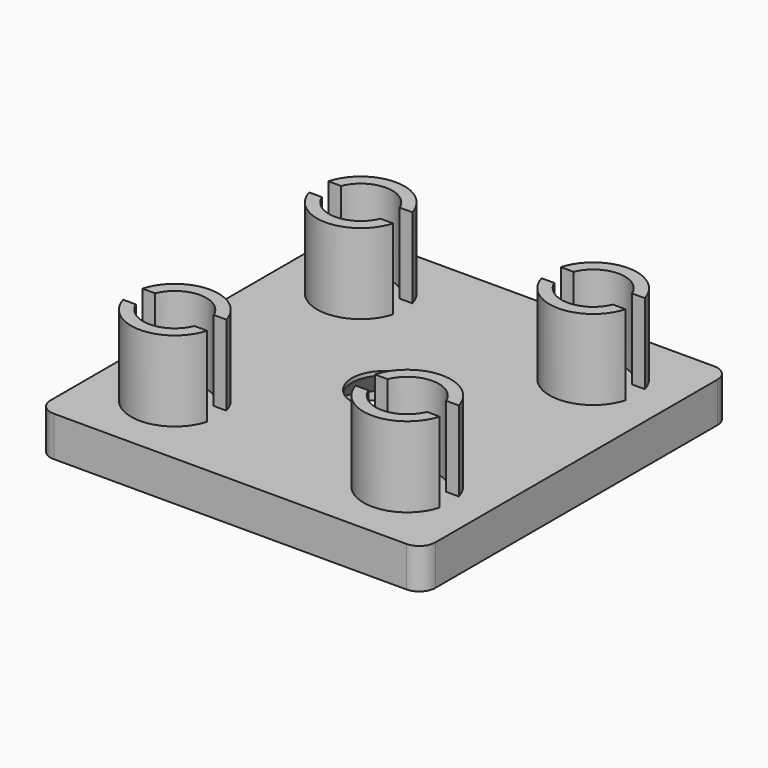
from build123d import *

# Parameters (mm, degrees)
F0_W           = 36
F0_H           = 36
F1_DEPTH       = 4
F3_DEPTH       = 10
F5_D           = 8
F5_CSINK_D     = 15
F5_CSINK_ANGLE = 90
F6_DEPTH       = 1


with BuildPart() as f1:
    # F0 (on Top) → F1 (new body)
    with BuildSketch(Plane.XY):
        with BuildLine():
            ThreePointArc((24, 22), (23.4142135624, 23.4142135624), (22, 24))
            Line((22, 24), (-22, 24))
            ThreePointArc((-22, 24), (-23.4142135624, 23.4142135624), (-24, 22))
            Line((-24, 22), (-24, -22))
            ThreePointArc((-24, -22), (-23.4142135624, -23.4142135624), (-22, -24))
            Line((-22, -24), (22, -24))
            ThreePointArc((22, -24), (23.4142135624, -23.4142135624), (24, -22))
            Line((24, -22), (24, 22))
        make_face()
        Rectangle(F0_W, F0_H, mode=Mode.SUBTRACT)
        Rectangle(F0_W, F0_H)
    extrude(amount=-F1_DEPTH)

    # F2 (on face) → F3 (join)
    with BuildSketch(Plane.XY):
        with BuildLine():
            Line((18.1541072781, 16), (19.7395133362, 16))
            ThreePointArc((19.7395133362, 16), (14.5, 19.95), (9.2604866638, 16))
            Line((9.2604866638, 16), (10.8458927219, 16))
            ThreePointArc((10.8458927219, 16), (14.5, 18.45), (18.1541072781, 16))
        make_face()
        with BuildLine():
            ThreePointArc((9.2604866638, 13), (14.5, 9.05), (19.7395133362, 13))
            Line((19.7395133362, 13), (18.1541072781, 13))
            ThreePointArc((18.1541072781, 13), (14.5, 10.55), (10.8458927219, 13))
            Line((10.8458927219, 13), (9.2604866638, 13))
        make_face()
        with BuildLine():
            Line((-10.8458927219, 16), (-9.2604866638, 16))
            ThreePointArc((-9.2604866638, 16), (-14.5, 19.95), (-19.7395133362, 16))
            Line((-19.7395133362, 16), (-18.1541072781, 16))
            ThreePointArc((-18.1541072781, 16), (-14.5, 18.45), (-10.8458927219, 16))
        make_face()
        with BuildLine():
            ThreePointArc((-19.7395133362, 13), (-14.5, 9.05), (-9.2604866638, 13))
            Line((-9.2604866638, 13), (-10.8458927219, 13))
            ThreePointArc((-10.8458927219, 13), (-14.5, 10.55), (-18.1541072781, 13))
            Line((-18.1541072781, 13), (-19.7395133362, 13))
        make_face()
        with BuildLine():
            Line((18.1541072781, -13), (19.7395133362, -13))
            ThreePointArc((19.7395133362, -13), (14.5, -9.05), (9.2604866638, -13))
            Line((9.2604866638, -13), (10.8458927219, -13))
            ThreePointArc((10.8458927219, -13), (14.5, -10.55), (18.1541072781, -13))
        make_face()
        with BuildLine():
            ThreePointArc((9.2604866638, -16), (14.5, -19.95), (19.7395133362, -16))
            Line((19.7395133362, -16), (18.1541072781, -16))
            ThreePointArc((18.1541072781, -16), (14.5, -18.45), (10.8458927219, -16))
            Line((10.8458927219, -16), (9.2604866638, -16))
        make_face()
        with BuildLine():
            ThreePointArc((-9.2604866638, -13), (-14.5, -9.05), (-19.7395133362, -13))
            Line((-19.7395133362, -13), (-18.1541072781, -13))
            ThreePointArc((-18.1541072781, -13), (-14.5, -10.55), (-10.8458927219, -13))
            Line((-10.8458927219, -13), (-9.2604866638, -13))
        make_face()
        with BuildLine():
            Line((-18.1541072781, -16), (-19.7395133362, -16))
            ThreePointArc((-19.7395133362, -16), (-14.5, -19.95), (-9.2604866638, -16))
            Line((-9.2604866638, -16), (-10.8458927219, -16))
            ThreePointArc((-10.8458927219, -16), (-14.5, -18.45), (-18.1541072781, -16))
        make_face()
    extrude(amount=F3_DEPTH)

    # F5 (through all)
    with Locations(Plane(origin=(0, 0, -4), x_dir=(1, 0, 0), z_dir=(0, 0, -1))):
        with Locations((0, 0)):
            CounterSinkHole(F5_D / 2, F5_CSINK_D / 2, counter_sink_angle=F5_CSINK_ANGLE)

    # F6 (add): a face of the model
    f6_faces = [f1.faces().sort_by_distance(p)[0] for p in [
        (22.9342135624, 22.9342135624, -4),
    ]]
    extrude(f6_faces, amount=F6_DEPTH)


solid = f1.part
